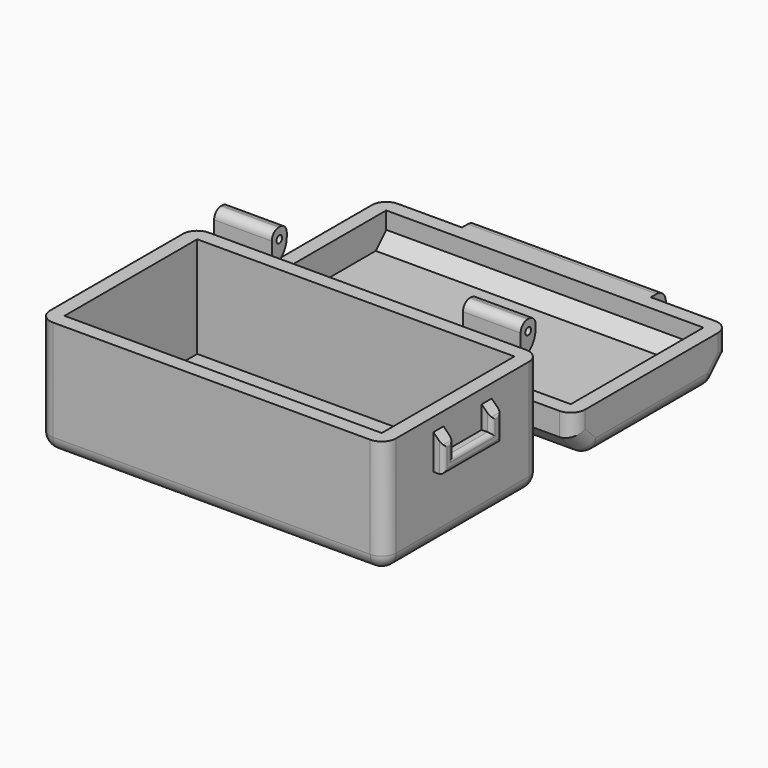
from build123d import *

# Parameters (mm, degrees)
F0_W           = 60.96
F0_H           = 34.29
F1_DEPTH       = 20.32
F2_T           = -2.54
F3_R           = 2.54
F4_W           = 60.96
F4_H           = 34.29
F5_DEPTH       = 7.874
F6_SIZE        = 3.81
F7_T           = -2.54
F8_W           = 10.16
F8_H           = 3.81
F8_H_2         = 2.032
F9_DEPTH       = 3.302
F10_R          = 2.54
F12_D          = 1.27
F14_DEPTH      = 3.7592
F15_W          = 14.5933912136
F15_H          = 2.2978205234
F16_DEPTH      = 25.4
F17_F1_R       = 1.524
F17_F2_R       = 1.524
F17_F3_R       = 1.524
F17_F4_R       = 1.524
F17_2_T1_DEPTH = 26.3766839159
F17_2_T3_DEPTH = 11.938
F19_T1_DEPTH   = 28.459343391
F19_T3_DEPTH   = 28.459343391
F18_W          = 33.274
F18_H          = 4.064
F20_DEPTH      = 3.302
F22_D          = 1.27
F23_R          = 2.023593808
F26_DEPTH      = 1.778
F27_SIZE       = 1.77799
F28_R          = 0.762
F29_DEPTH      = 1.778
F30_SIZE       = 1.77799
F31_R          = 0.762


# Not quite as in the source:
# - a fillet or chamfer that OpenCascade refuses, or shapes differently, is made with other operations: its cross-section is extruded or revolved along the edge and cut away or added
# - a fillet or chamfer is up to 0.001 mm smaller than in the source, because OpenCascade refuses the exact size


with BuildPart() as f1:
    # F0 (on Top) → F1 (new body)
    with BuildSketch(Plane.XY):
        Rectangle(F0_W, F0_H)
    extrude(amount=F1_DEPTH)

    # F2
    f2_openings = [f1.faces().sort_by_distance(p)[0] for p in [
        (0, 0, 20.32),
    ]]
    offset(amount=F2_T, openings=f2_openings)

    # F3
    f3_edges = [f1.edges().sort_by_distance(p)[0] for p in [
        (0, -17.145, 0),
        (-30.48, 0, 0),
        (0, 17.145, 0),
        (30.48, 0, 0),
        (-30.48, -17.145, 10.16),
        (-30.48, 17.145, 10.16),
        (30.48, 17.145, 10.16),
        (30.48, -17.145, 10.16),
    ]]
    fillet(f3_edges, radius=F3_R)

    # F8 (on face) → F9 (join)
    with BuildSketch(Plane(origin=(0, 17.145, 0), x_dir=(-1, 0, 0), z_dir=(0, 1, 0))):
        with Locations((21.9121703571, 22.225)):
            Rectangle(F8_W, F8_H)
        with Locations((21.9121703571, 19.304)):
            Rectangle(F8_W, F8_H_2)
        with Locations((-21.9202, 19.304)):
            Rectangle(F8_W, F8_H_2)
        with Locations((-21.9202, 22.225)):
            Rectangle(F8_W, F8_H)
    extrude(amount=F9_DEPTH)

    # F12 (through all)
    with Locations(Plane(origin=(-26.9921703571, 0, 0), x_dir=(0, -1, 0), z_dir=(-1, 0, 0))):
        with Locations((-18.796, 22.225)):
            Hole(F12_D / 2)

    # F17: fillet of radius 1.524 on 4 edges, made by hand

    # F17_f1
    f17_f1_edges = [f1.edges().sort_by_distance(p)[0] for p in [
        (21.9202, 17.145, 24.13),
    ]]
    fillet(f17_f1_edges, radius=F17_F1_R)

    # F17_f2
    f17_f2_edges = [f1.edges().sort_by_distance(p)[0] for p in [
        (-21.9121703571, 17.145, 24.13),
    ]]
    fillet(f17_f2_edges, radius=F17_F2_R)

    # F17_f3
    f17_f3_edges = [f1.edges().sort_by_distance(p)[0] for p in [
        (-21.9121703571, 20.447, 24.13),
    ]]
    fillet(f17_f3_edges, radius=F17_F3_R)

    # F17_f4
    f17_f4_edges = [f1.edges().sort_by_distance(p)[0] for p in [
        (21.9202, 20.447, 24.13),
    ]]
    fillet(f17_f4_edges, radius=F17_F4_R)

    # F19: fillet of radius 3.6792614691 on 2 edges, made by hand

    # F19_s2 → F19_t1 (cut)
    with BuildSketch(Plane.YZ.offset(-36.1418420526)):
        with BuildLine():
            ThreePointArc((17.145, 18.288), (19.4994969888, 19.4832265773), (20.447, 21.9478686782))
            Line((20.447, 21.9478686782), (20.447, 18.288))
            Line((20.447, 18.288), (17.145, 18.288))
        make_face()
    extrude(amount=F19_T1_DEPTH, mode=Mode.SUBTRACT)

    # F19_s4 → F19_t3 (cut)
    with BuildSketch(Plane.YZ.offset(7.6905283045)):
        with BuildLine():
            ThreePointArc((20.447, 21.9478686782), (19.4994969888, 19.4832265773), (17.145, 18.288))
            Line((17.145, 18.288), (20.447, 18.288))
            Line((20.447, 18.288), (20.447, 21.9478686782))
        make_face()
    extrude(amount=F19_T3_DEPTH, mode=Mode.SUBTRACT)

    # F25 (on face) → F26 (join)
    with BuildSketch(Plane(origin=(-30.48, 0, 0), x_dir=(0, -1, 0), z_dir=(-1, 0, 0))):
        Polygon((-4.1945250705, 18.0457551032), (-6.445246283, 18.0457551032), (-6.445246283, 11.6346105933), (6.5134512261, 11.6346105933), (6.5134512261, 18.0457551032), (4.12632199, 18.0457551032), (4.12632199, 14.0217393637), (-4.1945250705, 14.0217393637), align=None)
    extrude(amount=F26_DEPTH)

    # F27 (size 1.778 in the source; OpenCascade refuses exactly that, so slightly less here)
    f27_edges = [f1.edges().sort_by_distance(p)[0] for p in [
        (-32.258, 5.319886, 18.045755),
        (-32.258, -5.319887, 18.045755),
    ]]
    chamfer(f27_edges, length=F27_SIZE)

    # F28
    f28_edges = [f1.edges().sort_by_distance(p)[0] for p in [
        (-32.258, 6.445246, 13.951188),
        (-32.258, 5.319886, 16.267765),
        (-32.258, -0.034102, 11.634611),
        (-32.258, 4.194525, 15.144752),
        (-32.258, -6.513451, 13.951188),
        (-32.258, 0.034102, 14.021739),
        (-32.258, -5.319887, 16.267765),
        (-32.258, -4.126322, 15.144752),
    ]]
    fillet(f28_edges, radius=F28_R)

    # F24 (on face) → F29 (join)
    with BuildSketch(Plane.YZ.offset(30.48)):
        Polygon((-4.1808448732, 17.946805805), (-6.3891597092, 17.946805805), (-6.3891597092, 11.7778191343), (6.4262, 11.7778191343), (6.4262, 17.946805805), (4.2164, 17.946805805), (4.2164, 13.9876191343), (-4.1808448732, 13.9876191343), align=None)
    extrude(amount=F29_DEPTH)

    # F30 (size 1.778 in the source; OpenCascade refuses exactly that, so slightly less here)
    f30_edges = [f1.edges().sort_by_distance(p)[0] for p in [
        (32.258, -5.285002, 17.946806),
        (32.258, 5.3213, 17.946806),
    ]]
    chamfer(f30_edges, length=F30_SIZE)

    # F31
    f31_edges = [f1.edges().sort_by_distance(p)[0] for p in [
        (32.258, -6.38916, 13.973317),
        (32.258, -5.285002, 16.168816),
        (32.258, 0.01852, 11.777819),
        (32.258, -4.180845, 15.078217),
        (32.258, 6.4262, 13.973317),
        (32.258, 0.017778, 13.987619),
        (32.258, 5.3213, 16.168816),
        (32.258, 4.2164, 15.078217),
    ]]
    fillet(f31_edges, radius=F31_R)


with BuildPart() as f5:
    # F4 (on Top) → F5 (new body)
    with BuildSketch(Plane.XY):
        with Locations((0, 41.6224255873)):
            Rectangle(F4_W, F4_H)
    extrude(amount=F5_DEPTH)

    # F6
    f6_edges = [f5.edges().sort_by_distance(p)[0] for p in [
        (0, 58.767426, 0),
        (0, 24.477426, 0),
    ]]
    chamfer(f6_edges, length=F6_SIZE)

    # F7
    f7_openings = [f5.faces().sort_by_distance(p)[0] for p in [
        (0, 41.622426, 7.874),
    ]]
    offset(amount=F7_T, openings=f7_openings)

    # F10
    f10_edges = [f5.edges().sort_by_distance(p)[0] for p in [
        (0, 54.957426, 0),
        (0, 28.287426, 0),
        (30.48, 26.382426, 1.905),
        (30.48, 41.622426, 0),
        (30.48, 56.862426, 1.905),
        (-30.48, 56.862426, 1.905),
        (-30.48, 41.622426, 0),
        (-30.48, 58.767426, 5.842),
        (-30.48, 26.382426, 1.905),
        (-30.48, 24.477426, 5.842),
        (30.48, 24.477426, 5.842),
        (30.48, 58.767426, 5.842),
    ]]
    fillet(f10_edges, radius=F10_R)

    # F13 (on face) → F14 (join)
    with BuildSketch(Plane(origin=(0, 0, 0), x_dir=(1, 0, 0), z_dir=(0, 0, -1))):
        Polygon((-9.3783419579, -43.7814255873), (0, -43.7814255873), (9.3783419579, -43.7814255873), (9.3783419579, -39.4634255873), (-9.3783419579, -39.4634255873), align=None)
    extrude(amount=F14_DEPTH)

    # F15 (on face) → F16 (cut)
    with BuildSketch(Plane.XZ.offset(-39.4634255873)):
        with Locations((-0.1355621498, -1.1489102617)):
            Rectangle(F15_W, F15_H)
    extrude(amount=-F16_DEPTH, mode=Mode.SUBTRACT)

    # F17#2: fillet of radius 1.524 on 4 edges, made by hand

    # F17_2_s2 → F17_2_t1 (cut)
    with BuildSketch(Plane.YZ.offset(-13.1883419579)):
        with BuildLine():
            ThreePointArc((42.2574255873, -3.7592), (43.3350563218, -3.3128307345), (43.7814255873, -2.2352))
            Line((43.7814255873, -2.2352), (43.7814255873, -3.7592))
            Line((43.7814255873, -3.7592), (42.2574255873, -3.7592))
        make_face()
        with BuildLine():
            ThreePointArc((40.9874255873, -3.7592), (39.9097948527, -3.3128307345), (39.4634255873, -2.2352))
            Line((39.4634255873, -2.2352), (39.4634255873, -3.7592))
            Line((39.4634255873, -3.7592), (40.9874255873, -3.7592))
        make_face()
    extrude(amount=F17_2_T1_DEPTH, mode=Mode.SUBTRACT)

    # F17_2_s4 → F17_2_t3 (cut)
    with BuildSketch(Plane.XZ.offset(-47.5914255873)):
        with BuildLine():
            ThreePointArc((9.3783419579, -2.2352), (8.9319726925, -3.3128307345), (7.8543419579, -3.7592))
            Line((7.8543419579, -3.7592), (9.3783419579, -3.7592))
            Line((9.3783419579, -3.7592), (9.3783419579, -2.2352))
        make_face()
        with BuildLine():
            ThreePointArc((-7.8543419579, -3.7592), (-8.9319726925, -3.3128307345), (-9.3783419579, -2.2352))
            Line((-9.3783419579, -2.2352), (-9.3783419579, -3.7592))
            Line((-9.3783419579, -3.7592), (-7.8543419579, -3.7592))
        make_face()
    extrude(amount=F17_2_T3_DEPTH, mode=Mode.SUBTRACT)

    # F18 (on face) → F20 (join)
    with BuildSketch(Plane(origin=(0, 58.7674255873, 0), x_dir=(-1, 0, 0), z_dir=(0, 1, 0))):
        with Locations((0, 5.842)):
            Rectangle(F18_W, F18_H)
    extrude(amount=F20_DEPTH)

    # F22 (through all)
    with Locations(Plane(origin=(-16.637, 0, 0), x_dir=(0, -1, 0), z_dir=(-1, 0, 0))):
        with Locations((-60.4184255873, 5.842)):
            Hole(F22_D / 2)

    # F23
    f23_edges = [f5.edges().sort_by_distance(p)[0] for p in [
        (0, 62.069426, 7.874),
        (0, 62.069426, 3.81),
    ]]
    fillet(f23_edges, radius=F23_R)


solid = Compound([f1.part, f5.part])
